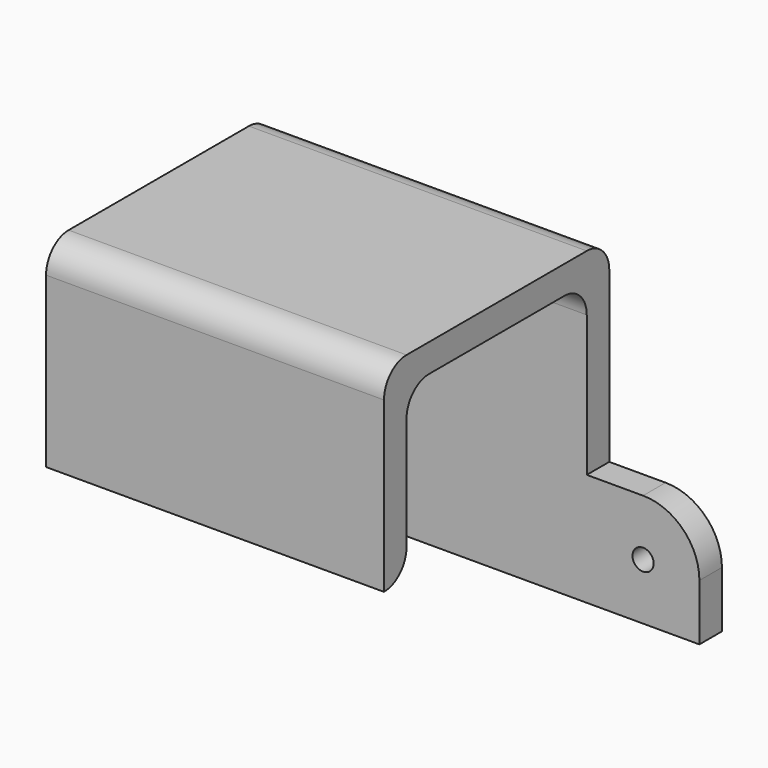
from build123d import *

# Parameters (mm, degrees)
F1_DEPTH = 6.35
F2_R     = 12.7
F4_DEPTH = 38.1
F5_R     = 6.34999


# Not quite as in the source:
# - a fillet or chamfer is up to 0.001 mm smaller than in the source, because OpenCascade refuses the exact size


with BuildPart() as f1:
    # F0 (on Front) → F1 (new body)
    with BuildSketch(Plane.XZ):
        with BuildLine():
            Line((63.5, 0), (63.5, 12.7))
            Line((63.5, 12.7), (-63.5, 12.7))
            Line((-63.5, 12.7), (-63.5, 0))
            Line((-63.5, 0), (-53.18125, 0))
            ThreePointArc((-53.18125, 0), (-50.8, 2.38125), (-48.41875, 0))
            Line((-48.41875, 0), (48.41875, 0))
            ThreePointArc((48.41875, 0), (50.8, 2.38125), (53.18125, 0))
            Line((53.18125, 0), (63.5, 0))
        make_face()
        with BuildLine():
            Line((63.5, -12.7), (63.5, 0))
            Line((63.5, 0), (53.18125, 0))
            ThreePointArc((53.18125, 0), (50.8, -2.38125), (48.41875, 0))
            Line((48.41875, 0), (-48.41875, 0))
            ThreePointArc((-48.41875, 0), (-50.8, -2.38125), (-53.18125, 0))
            Line((-53.18125, 0), (-63.5, 0))
            Line((-63.5, 0), (-63.5, -12.7))
            Line((-63.5, -12.7), (63.5, -12.7))
        make_face()
    extrude(amount=F1_DEPTH)

    # F2
    f2_edges = [f1.edges().sort_by_distance(p)[0] for p in [
        (-63.5, -3.175, 12.7),
        (63.5, -3.175, 12.7),
    ]]
    fillet(f2_edges, radius=F2_R)

    # F3 (on Right) → F4 (join, symmetric)
    with BuildSketch(Plane.YZ):
        Polygon((0, 12.7), (0, 57.15), (-63.5, 57.15), (-63.5, 12.7), (-57.15, 12.7), (-57.15, 50.8), (-6.35, 50.8), (-6.35, 12.7), align=None)
    extrude(amount=F4_DEPTH, both=True)

    # F5 (radius 6.35 in the source; OpenCascade refuses exactly that, so slightly less here)
    f5_edges = [f1.edges().sort_by_distance(p)[0] for p in [
        (0, 0, 57.15),
        (0, -63.5, 57.15),
        (0, -6.35, 50.8),
        (0, -57.15, 50.8),
        (0, -57.15, 12.7),
    ]]
    fillet(f5_edges, radius=F5_R)


solid = f1.part
